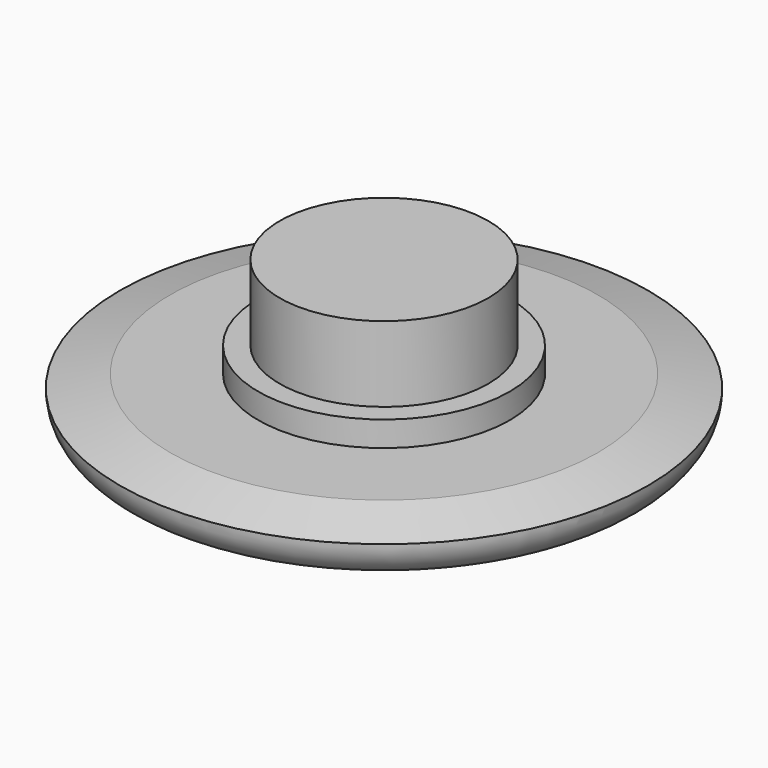
from build123d import *

# Parameters (mm, degrees)
F0_R     = 10.5
F1_DEPTH = 2
F2_R     = 5
F3_DEPTH = 1
F4_R     = 4.15
F5_DEPTH = 3
F6_SIZE2 = 0.5
F6_SIZE  = 2
F7_R     = 1.49999


# Not quite as in the source:
# - a fillet or chamfer is up to 0.001 mm smaller than in the source, because OpenCascade refuses the exact size


with BuildPart() as f1:
    # F0 (on Top) → F1 (new body)
    with BuildSketch(Plane.XY):
        Circle(F0_R)
    extrude(amount=F1_DEPTH)

    # F2 (on face) → F3 (join)
    with BuildSketch(Plane.XY.offset(2)):
        Circle(F2_R)
    extrude(amount=F3_DEPTH)

    # F4 (on face) → F5 (join)
    with BuildSketch(Plane.XY.offset(3)):
        Circle(F4_R)
    extrude(amount=F5_DEPTH)

    # F6
    f6_edges = [f1.edges().sort_by_distance(p)[0] for p in [
        (-10.5, 0, 2),
    ]]
    f6_side = f1.faces().sort_by_distance((-10.203015, 0, 2))[0]
    chamfer(f6_edges, length=F6_SIZE, length2=F6_SIZE2, reference=f6_side)

    # F7 (radius 1.5 in the source; OpenCascade refuses exactly that, so slightly less here)
    f7_edges = [f1.edges().sort_by_distance(p)[0] for p in [
        (-10.5, 0, 0),
    ]]
    fillet(f7_edges, radius=F7_R)


solid = f1.part
